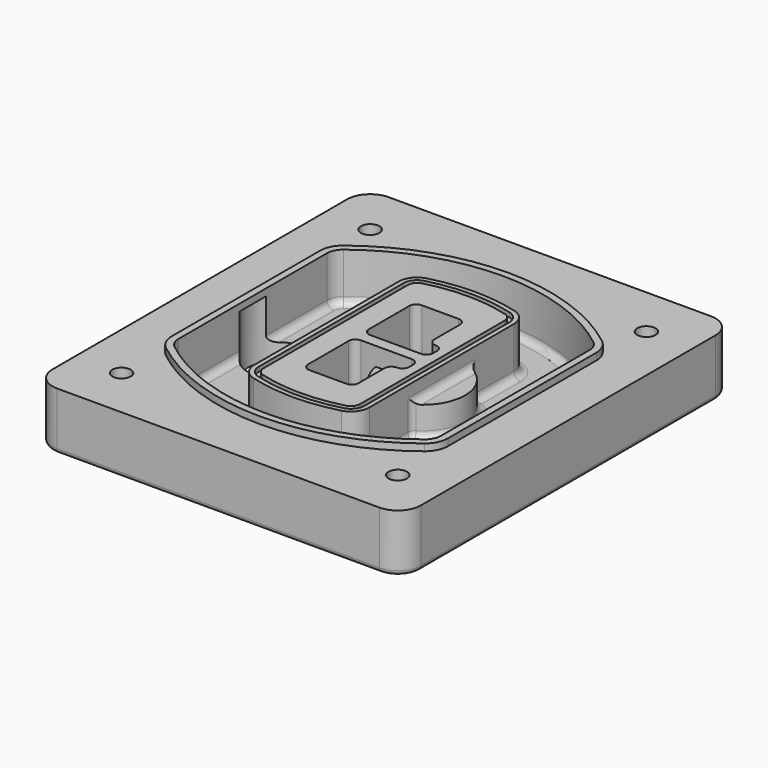
from build123d import *

# Parameters (mm, degrees)
F0_R      = 4
F1_DEPTH  = 25
F2_DEPTH  = 3
F3_DEPTH  = 18
F5_DEPTH  = 21
F6_DEPTH  = 2
F8_DEPTH  = 20
F9_DEPTH  = 16
F10_DEPTH = 25
F7_R      = 6
F7_R_2    = 4
F11_DEPTH = 6
F13_DEPTH = 9
F14_R     = 3
F15_R     = 2


# Not quite as in the source:
# - a feature of the source that left no trace in its solid (it failed there, or was rolled back) is left out


with BuildPart() as f1:
    # F0 (on Top) → F1 (new body)
    with BuildSketch(Plane.XY):
        with BuildLine():
            ThreePointArc((-80, -80), (-77.0710678119, -87.0710678119), (-70, -90))
            Line((-70, -90), (70, -90))
            ThreePointArc((70, -90), (77.0710678119, -87.0710678119), (80, -80))
            Line((80, -80), (80, 80))
            ThreePointArc((80, 80), (77.0710678119, 87.0710678119), (70, 90))
            Line((70, 90), (-70, 90))
            ThreePointArc((-70, 90), (-77.0710678119, 87.0710678119), (-80, 80))
            Line((-80, 80), (-80, -80))
        make_face()
        with Locations((-60, -67.5)):
            Circle(F0_R, mode=Mode.SUBTRACT)
        with Locations((60, -67.5)):
            Circle(F0_R, mode=Mode.SUBTRACT)
        with Locations((-60, 67.5)):
            Circle(F0_R, mode=Mode.SUBTRACT)
        with BuildLine():
            ThreePointArc((-64, 40.2934422872), (-62.5820384798, 46.4328484224), (-58.6153846154, 51.3286200352))
            ThreePointArc((-58.6153846154, 51.3286200352), (0, 71.5), (58.6153846154, 51.3286200352))
            ThreePointArc((58.6153846154, 51.3286200352), (62.5820384798, 46.4328484224), (64, 40.2934422872))
            Line((64, 40.2934422872), (64, -40.2934422872))
            ThreePointArc((64, -40.2934422872), (62.5820384798, -46.4328484224), (58.6153846154, -51.3286200352))
            ThreePointArc((58.6153846154, -51.3286200352), (0, -71.5), (-58.6153846154, -51.3286200352))
            ThreePointArc((-58.6153846154, -51.3286200352), (-62.5820384798, -46.4328484224), (-64, -40.2934422872))
            Line((-64, -40.2934422872), (-64, 40.2934422872))
        make_face(mode=Mode.SUBTRACT)
        with Locations((60, 67.5)):
            Circle(F0_R, mode=Mode.SUBTRACT)
        with BuildLine():
            ThreePointArc((58.6153846154, 51.3286200352), (0, 71.5), (-58.6153846154, 51.3286200352))
            ThreePointArc((-58.6153846154, 51.3286200352), (-62.5820384798, 46.4328484224), (-64, 40.2934422872))
            Line((-64, 40.2934422872), (-64, -40.2934422872))
            ThreePointArc((-64, -40.2934422872), (-62.5820384798, -46.4328484224), (-58.6153846154, -51.3286200352))
            ThreePointArc((-58.6153846154, -51.3286200352), (0, -71.5), (58.6153846154, -51.3286200352))
            ThreePointArc((58.6153846154, -51.3286200352), (62.5820384798, -46.4328484224), (64, -40.2934422872))
            Line((64, -40.2934422872), (64, 40.2934422872))
            ThreePointArc((64, 40.2934422872), (62.5820384798, 46.4328484224), (58.6153846154, 51.3286200352))
        make_face()
        with BuildLine():
            Line((-60, -40.2934422872), (-60, 40.2934422872))
            ThreePointArc((-60, 40.2934422872), (-58.9871703427, 44.6787323838), (-56.1538461538, 48.1757121072))
            ThreePointArc((-56.1538461538, 48.1757121072), (0, 67.5), (56.1538461538, 48.1757121072))
            ThreePointArc((56.1538461538, 48.1757121072), (58.9871703427, 44.6787323838), (60, 40.2934422872))
            Line((60, 40.2934422872), (60, -40.2934422872))
            ThreePointArc((60, -40.2934422872), (58.9871703427, -44.6787323838), (56.1538461538, -48.1757121072))
            ThreePointArc((56.1538461538, -48.1757121072), (0, -67.5), (-56.1538461538, -48.1757121072))
            ThreePointArc((-56.1538461538, -48.1757121072), (-58.9871703427, -44.6787323838), (-60, -40.2934422872))
        make_face(mode=Mode.SUBTRACT)
        with BuildLine():
            ThreePointArc((-56.1538461538, 48.1757121072), (-58.9871703427, 44.6787323838), (-60, 40.2934422872))
            Line((-60, 40.2934422872), (-60, -40.2934422872))
            ThreePointArc((-60, -40.2934422872), (-58.9871703427, -44.6787323838), (-56.1538461538, -48.1757121072))
            ThreePointArc((-56.1538461538, -48.1757121072), (0, -67.5), (56.1538461538, -48.1757121072))
            ThreePointArc((56.1538461538, -48.1757121072), (58.9871703427, -44.6787323838), (60, -40.2934422872))
            Line((60, -40.2934422872), (60, 40.2934422872))
            ThreePointArc((60, 40.2934422872), (58.9871703427, 44.6787323838), (56.1538461538, 48.1757121072))
            ThreePointArc((56.1538461538, 48.1757121072), (0, 67.5), (-56.1538461538, 48.1757121072))
        make_face()
        with BuildLine():
            ThreePointArc((54.3076923077, 45.8110311612), (56.2910192399, 43.3631453548), (57, 40.2934422872))
            Line((57, 40.2934422872), (57, -40.2934422872))
            ThreePointArc((57, -40.2934422872), (56.2910192399, -43.3631453548), (54.3076923077, -45.8110311612))
            ThreePointArc((54.3076923077, -45.8110311612), (0, -64.5), (-54.3076923077, -45.8110311612))
            ThreePointArc((-54.3076923077, -45.8110311612), (-56.2910192399, -43.3631453548), (-57, -40.2934422872))
            Line((-57, -40.2934422872), (-57, 40.2934422872))
            ThreePointArc((-57, 40.2934422872), (-56.2910192399, 43.3631453548), (-54.3076923077, 45.8110311612))
            ThreePointArc((-54.3076923077, 45.8110311612), (0, 64.5), (54.3076923077, 45.8110311612))
        make_face(mode=Mode.SUBTRACT)
        with BuildLine():
            Line((57, -40.2934422872), (57, 40.2934422872))
            ThreePointArc((57, 40.2934422872), (56.2910192399, 43.3631453548), (54.3076923077, 45.8110311612))
            ThreePointArc((54.3076923077, 45.8110311612), (0, 64.5), (-54.3076923077, 45.8110311612))
            ThreePointArc((-54.3076923077, 45.8110311612), (-56.2910192399, 43.3631453548), (-57, 40.2934422872))
            Line((-57, 40.2934422872), (-57, -40.2934422872))
            ThreePointArc((-57, -40.2934422872), (-56.2910192399, -43.3631453548), (-54.3076923077, -45.8110311612))
            ThreePointArc((-54.3076923077, -45.8110311612), (0, -64.5), (54.3076923077, -45.8110311612))
            ThreePointArc((54.3076923077, -45.8110311612), (56.2910192399, -43.3631453548), (57, -40.2934422872))
        make_face()
    extrude(amount=-F1_DEPTH)

    # F0 (on Top) → F2 (join)
    with BuildSketch(Plane.XY):
        with BuildLine():
            ThreePointArc((-56.1538461538, 48.1757121072), (-58.9871703427, 44.6787323838), (-60, 40.2934422872))
            Line((-60, 40.2934422872), (-60, -40.2934422872))
            ThreePointArc((-60, -40.2934422872), (-58.9871703427, -44.6787323838), (-56.1538461538, -48.1757121072))
            ThreePointArc((-56.1538461538, -48.1757121072), (0, -67.5), (56.1538461538, -48.1757121072))
            ThreePointArc((56.1538461538, -48.1757121072), (58.9871703427, -44.6787323838), (60, -40.2934422872))
            Line((60, -40.2934422872), (60, 40.2934422872))
            ThreePointArc((60, 40.2934422872), (58.9871703427, 44.6787323838), (56.1538461538, 48.1757121072))
            ThreePointArc((56.1538461538, 48.1757121072), (0, 67.5), (-56.1538461538, 48.1757121072))
        make_face()
        with BuildLine():
            ThreePointArc((54.3076923077, 45.8110311612), (56.2910192399, 43.3631453548), (57, 40.2934422872))
            Line((57, 40.2934422872), (57, -40.2934422872))
            ThreePointArc((57, -40.2934422872), (56.2910192399, -43.3631453548), (54.3076923077, -45.8110311612))
            ThreePointArc((54.3076923077, -45.8110311612), (0, -64.5), (-54.3076923077, -45.8110311612))
            ThreePointArc((-54.3076923077, -45.8110311612), (-56.2910192399, -43.3631453548), (-57, -40.2934422872))
            Line((-57, -40.2934422872), (-57, 40.2934422872))
            ThreePointArc((-57, 40.2934422872), (-56.2910192399, 43.3631453548), (-54.3076923077, 45.8110311612))
            ThreePointArc((-54.3076923077, 45.8110311612), (0, 64.5), (54.3076923077, 45.8110311612))
        make_face(mode=Mode.SUBTRACT)
    extrude(amount=F2_DEPTH)

    # F0 (on Top) → F3 (cut)
    with BuildSketch(Plane.XY):
        with BuildLine():
            Line((57, -40.2934422872), (57, 40.2934422872))
            ThreePointArc((57, 40.2934422872), (56.2910192399, 43.3631453548), (54.3076923077, 45.8110311612))
            ThreePointArc((54.3076923077, 45.8110311612), (0, 64.5), (-54.3076923077, 45.8110311612))
            ThreePointArc((-54.3076923077, 45.8110311612), (-56.2910192399, 43.3631453548), (-57, 40.2934422872))
            Line((-57, 40.2934422872), (-57, -40.2934422872))
            ThreePointArc((-57, -40.2934422872), (-56.2910192399, -43.3631453548), (-54.3076923077, -45.8110311612))
            ThreePointArc((-54.3076923077, -45.8110311612), (0, -64.5), (54.3076923077, -45.8110311612))
            ThreePointArc((54.3076923077, -45.8110311612), (56.2910192399, -43.3631453548), (57, -40.2934422872))
        make_face()
    extrude(amount=-F3_DEPTH, mode=Mode.SUBTRACT)

    # F4 (on face) → F5 (join, through all)
    with BuildSketch(Plane.XY.offset(3)):
        with BuildLine():
            ThreePointArc((-25, -39.2465276821), (-23.3511545998, -44.1109737193), (-19.0842911877, -46.9702398883))
            ThreePointArc((-19.0842911877, -46.9702398883), (0, -49.5), (19.0842911877, -46.9702398883))
            ThreePointArc((19.0842911877, -46.9702398883), (23.3511545998, -44.1109737193), (25, -39.2465276821))
            Line((25, -39.2465276821), (25, 39.2465276821))
            ThreePointArc((25, 39.2465276821), (23.3511545998, 44.1109737193), (19.0842911877, 46.9702398883))
            ThreePointArc((19.0842911877, 46.9702398883), (0, 49.5), (-19.0842911877, 46.9702398883))
            ThreePointArc((-19.0842911877, 46.9702398883), (-23.3511545998, 44.1109737193), (-25, 39.2465276821))
            Line((-25, 39.2465276821), (-25, -39.2465276821))
        make_face()
        with BuildLine():
            ThreePointArc((18.5632183908, 45.0393118368), (21.7633659499, 42.89486221), (23, 39.2465276821))
            Line((23, 39.2465276821), (23, -39.2465276821))
            ThreePointArc((23, -39.2465276821), (21.7633659499, -42.89486221), (18.5632183908, -45.0393118368))
            ThreePointArc((18.5632183908, -45.0393118368), (0, -47.5), (-18.5632183908, -45.0393118368))
            ThreePointArc((-18.5632183908, -45.0393118368), (-21.7633659499, -42.89486221), (-23, -39.2465276821))
            Line((-23, -39.2465276821), (-23, 39.2465276821))
            ThreePointArc((-23, 39.2465276821), (-21.7633659499, 42.89486221), (-18.5632183908, 45.0393118368))
            ThreePointArc((-18.5632183908, 45.0393118368), (0, 47.5), (18.5632183908, 45.0393118368))
        make_face(mode=Mode.SUBTRACT)
        with BuildLine():
            Line((23, -39.2465276821), (23, 39.2465276821))
            ThreePointArc((23, 39.2465276821), (21.7633659499, 42.89486221), (18.5632183908, 45.0393118368))
            ThreePointArc((18.5632183908, 45.0393118368), (0, 47.5), (-18.5632183908, 45.0393118368))
            ThreePointArc((-18.5632183908, 45.0393118368), (-21.7633659499, 42.89486221), (-23, 39.2465276821))
            Line((-23, 39.2465276821), (-23, -39.2465276821))
            ThreePointArc((-23, -39.2465276821), (-21.7633659499, -42.89486221), (-18.5632183908, -45.0393118368))
            ThreePointArc((-18.5632183908, -45.0393118368), (0, -47.5), (18.5632183908, -45.0393118368))
            ThreePointArc((18.5632183908, -45.0393118368), (21.7633659499, -42.89486221), (23, -39.2465276821))
        make_face()
        with BuildLine():
            ThreePointArc((18.0421455939, 43.1083837852), (20.1755772999, 41.6787507007), (21, 39.2465276821))
            Line((21, 39.2465276821), (21, -39.2465276821))
            ThreePointArc((21, -39.2465276821), (20.1755772999, -41.6787507007), (18.0421455939, -43.1083837852))
            ThreePointArc((18.0421455939, -43.1083837852), (0, -45.5), (-18.0421455939, -43.1083837852))
            ThreePointArc((-18.0421455939, -43.1083837852), (-20.1755772999, -41.6787507007), (-21, -39.2465276821))
            Line((-21, -39.2465276821), (-21, 39.2465276821))
            ThreePointArc((-21, 39.2465276821), (-20.1755772999, 41.6787507007), (-18.0421455939, 43.1083837852))
            ThreePointArc((-18.0421455939, 43.1083837852), (0, 45.5), (18.0421455939, 43.1083837852))
        make_face(mode=Mode.SUBTRACT)
        with BuildLine():
            Line((21, -39.2465276821), (21, 39.2465276821))
            ThreePointArc((21, 39.2465276821), (20.1755772999, 41.6787507007), (18.0421455939, 43.1083837852))
            ThreePointArc((18.0421455939, 43.1083837852), (0, 45.5), (-18.0421455939, 43.1083837852))
            ThreePointArc((-18.0421455939, 43.1083837852), (-20.1755772999, 41.6787507007), (-21, 39.2465276821))
            Line((-21, 39.2465276821), (-21, -39.2465276821))
            ThreePointArc((-21, -39.2465276821), (-20.1755772999, -41.6787507007), (-18.0421455939, -43.1083837852))
            ThreePointArc((-18.0421455939, -43.1083837852), (0, -45.5), (18.0421455939, -43.1083837852))
            ThreePointArc((18.0421455939, -43.1083837852), (20.1755772999, -41.6787507007), (21, -39.2465276821))
        make_face()
        with BuildLine():
            Line((-8, -2.5), (14, -2.5))
            ThreePointArc((14, -2.5), (16.1213203436, -3.3786796564), (17, -5.5))
            Line((17, -5.5), (17, -7.5))
            ThreePointArc((17, -7.5), (16.1213203436, -9.6213203436), (14, -10.5))
            ThreePointArc((14, -10.5), (11.8786796564, -11.3786796564), (11, -13.5))
            Line((11, -13.5), (11, -27.5))
            ThreePointArc((11, -27.5), (10.1213203436, -29.6213203436), (8, -30.5))
            Line((8, -30.5), (-8, -30.5))
            ThreePointArc((-8, -30.5), (-10.1213203436, -29.6213203436), (-11, -27.5))
            Line((-11, -27.5), (-11, -5.5))
            ThreePointArc((-11, -5.5), (-10.1213203436, -3.3786796564), (-8, -2.5))
        make_face(mode=Mode.SUBTRACT)
        with BuildLine():
            ThreePointArc((-8, 2.5), (-10.1213203436, 3.3786796564), (-11, 5.5))
            Line((-11, 5.5), (-11, 27.5))
            ThreePointArc((-11, 27.5), (-10.1213203436, 29.6213203436), (-8, 30.5))
            Line((-8, 30.5), (8, 30.5))
            ThreePointArc((8, 30.5), (10.1213203436, 29.6213203436), (11, 27.5))
            Line((11, 27.5), (11, 13.5))
            ThreePointArc((11, 13.5), (11.8786796564, 11.3786796564), (14, 10.5))
            ThreePointArc((14, 10.5), (16.1213203436, 9.6213203436), (17, 7.5))
            Line((17, 7.5), (17, 5.5))
            ThreePointArc((17, 5.5), (16.1213203436, 3.3786796564), (14, 2.5))
            Line((14, 2.5), (-8, 2.5))
        make_face(mode=Mode.SUBTRACT)
    extrude(amount=-F5_DEPTH)

    # F4 (on face) → F6 (cut)
    with BuildSketch(Plane.XY.offset(3)):
        with BuildLine():
            Line((23, -39.2465276821), (23, 39.2465276821))
            ThreePointArc((23, 39.2465276821), (21.7633659499, 42.89486221), (18.5632183908, 45.0393118368))
            ThreePointArc((18.5632183908, 45.0393118368), (0, 47.5), (-18.5632183908, 45.0393118368))
            ThreePointArc((-18.5632183908, 45.0393118368), (-21.7633659499, 42.89486221), (-23, 39.2465276821))
            Line((-23, 39.2465276821), (-23, -39.2465276821))
            ThreePointArc((-23, -39.2465276821), (-21.7633659499, -42.89486221), (-18.5632183908, -45.0393118368))
            ThreePointArc((-18.5632183908, -45.0393118368), (0, -47.5), (18.5632183908, -45.0393118368))
            ThreePointArc((18.5632183908, -45.0393118368), (21.7633659499, -42.89486221), (23, -39.2465276821))
        make_face()
        with BuildLine():
            ThreePointArc((18.0421455939, 43.1083837852), (20.1755772999, 41.6787507007), (21, 39.2465276821))
            Line((21, 39.2465276821), (21, -39.2465276821))
            ThreePointArc((21, -39.2465276821), (20.1755772999, -41.6787507007), (18.0421455939, -43.1083837852))
            ThreePointArc((18.0421455939, -43.1083837852), (0, -45.5), (-18.0421455939, -43.1083837852))
            ThreePointArc((-18.0421455939, -43.1083837852), (-20.1755772999, -41.6787507007), (-21, -39.2465276821))
            Line((-21, -39.2465276821), (-21, 39.2465276821))
            ThreePointArc((-21, 39.2465276821), (-20.1755772999, 41.6787507007), (-18.0421455939, 43.1083837852))
            ThreePointArc((-18.0421455939, 43.1083837852), (0, 45.5), (18.0421455939, 43.1083837852))
        make_face(mode=Mode.SUBTRACT)
    extrude(amount=-F6_DEPTH, mode=Mode.SUBTRACT)

    # F7 (on face) → F8 (join)
    with BuildSketch(Plane(origin=(0, 0, -25), x_dir=(1, 0, 0), z_dir=(0, 0, -1))):
        with BuildLine():
            ThreePointArc((3.28842436, 0), (16.7567035675, 13.4682792075), (30.224982775, 0))
            Line((30.224982775, 0), (35.224982775, 0))
            ThreePointArc((35.224982775, 0), (16.7567035675, 18.4682792075), (-1.71157564, 0))
            Line((-1.71157564, 0), (3.28842436, 0))
        make_face()
        with BuildLine():
            Line((3.28842436, 0), (30.224982775, 0))
            ThreePointArc((30.224982775, 0), (16.7567035675, 13.4682792075), (3.28842436, 0))
        make_face()
        with BuildLine():
            ThreePointArc((3.28842436, 0), (16.7567035675, -13.4682792075), (30.224982775, 0))
            Line((30.224982775, 0), (3.28842436, 0))
        make_face()
        with BuildLine():
            Line((35.224982775, 0), (30.224982775, 0))
            ThreePointArc((30.224982775, 0), (16.7567035675, -13.4682792075), (3.28842436, 0))
            Line((3.28842436, 0), (-1.71157564, 0))
            ThreePointArc((-1.71157564, 0), (16.7567035675, -18.4682792075), (35.224982775, 0))
        make_face()
    extrude(amount=-F8_DEPTH)

    # F7 (on face) → F9 (cut)
    with BuildSketch(Plane(origin=(0, 0, -25), x_dir=(1, 0, 0), z_dir=(0, 0, -1))):
        with BuildLine():
            Line((3.28842436, 0), (30.224982775, 0))
            ThreePointArc((30.224982775, 0), (16.7567035675, 13.4682792075), (3.28842436, 0))
        make_face()
        with BuildLine():
            ThreePointArc((3.28842436, 0), (16.7567035675, -13.4682792075), (30.224982775, 0))
            Line((30.224982775, 0), (3.28842436, 0))
        make_face()
    extrude(amount=-F9_DEPTH, mode=Mode.SUBTRACT)

    # F7 (on face) → F10 (cut)
    with BuildSketch(Plane(origin=(0, 0, -25), x_dir=(1, 0, 0), z_dir=(0, 0, -1))):
        with BuildLine():
            Line((-59.0318229325, 0), (-32.0952645175, 0))
            ThreePointArc((-32.0952645175, 0), (-45.563543725, 13.4682792075), (-59.0318229325, 0))
        make_face()
        with BuildLine():
            ThreePointArc((-59.0318229325, 0), (-45.563543725, -13.4682792075), (-32.0952645175, 0))
            Line((-32.0952645175, 0), (-59.0318229325, 0))
        make_face()
    extrude(amount=-F10_DEPTH, mode=Mode.SUBTRACT)

    # F7 (on face) → F11 (cut)
    with BuildSketch(Plane(origin=(0, 0, -25), x_dir=(1, 0, 0), z_dir=(0, 0, -1))):
        with Locations((60, -67.5)):
            Circle(F7_R)
        with Locations((60, -67.5)):
            Circle(F7_R_2, mode=Mode.SUBTRACT)
        with Locations((-60, -67.5)):
            Circle(F7_R)
        with Locations((-60, -67.5)):
            Circle(F7_R_2, mode=Mode.SUBTRACT)
        with Locations((-60, 67.5)):
            Circle(F7_R)
        with Locations((-60, 67.5)):
            Circle(F7_R_2, mode=Mode.SUBTRACT)
        with Locations((60, 67.5)):
            Circle(F7_R)
        with Locations((60, 67.5)):
            Circle(F7_R_2, mode=Mode.SUBTRACT)
    extrude(amount=-F11_DEPTH, mode=Mode.SUBTRACT)

    # F12 (on face) → F13 (cut, through all)
    with BuildSketch(Plane(origin=(0, 0, -9), x_dir=(1, 0, 0), z_dir=(0, 0, -1))):
        with BuildLine():
            Line((11, 13.5), (11, 17.5481537753))
            ThreePointArc((11, 17.5481537753), (2.5696536419, 11.8239143813), (-1.5415842455, 2.5))
            Line((-1.5415842455, 2.5), (3.5224848595, 2.5))
            ThreePointArc((3.5224848595, 2.5), (6.1857188154, 8.3455872281), (11.2536447004, 12.2927168648))
            ThreePointArc((11.2536447004, 12.2927168648), (11.0640958889, 12.8831798879), (11, 13.5))
        make_face()
        with BuildLine():
            ThreePointArc((11.2536447004, -12.2927168648), (6.1857188154, -8.3455872281), (3.5224848595, -2.5))
            Line((3.5224848595, -2.5), (-1.5415842455, -2.5))
            ThreePointArc((-1.5415842455, -2.5), (2.5696536419, -11.8239143813), (11, -17.5481537753))
            Line((11, -17.5481537753), (11, -13.5))
            ThreePointArc((11, -13.5), (11.0640958889, -12.8831798879), (11.2536447004, -12.2927168648))
        make_face()
        with BuildLine():
            ThreePointArc((11.2536447004, 12.2927168648), (6.1857188154, 8.3455872281), (3.5224848595, 2.5))
            Line((3.5224848595, 2.5), (14, 2.5))
            ThreePointArc((14, 2.5), (16.1213203436, 3.3786796564), (17, 5.5))
            Line((17, 5.5), (17, 7.5))
            ThreePointArc((17, 7.5), (16.1213203436, 9.6213203436), (14, 10.5))
            ThreePointArc((14, 10.5), (12.3601599782, 10.9878446101), (11.2536447004, 12.2927168648))
        make_face()
        with BuildLine():
            Line((14, -2.5), (3.5224848595, -2.5))
            ThreePointArc((3.5224848595, -2.5), (6.1857188154, -8.3455872281), (11.2536447004, -12.2927168648))
            ThreePointArc((11.2536447004, -12.2927168648), (12.3601599782, -10.9878446101), (14, -10.5))
            ThreePointArc((14, -10.5), (16.1213203436, -9.6213203436), (17, -7.5))
            Line((17, -7.5), (17, -5.5))
            ThreePointArc((17, -5.5), (16.1213203436, -3.3786796564), (14, -2.5))
        make_face()
    extrude(amount=F13_DEPTH, mode=Mode.SUBTRACT)

    # F14
    f14_edges = [f1.edges().sort_by_distance(p)[0] for p in [
        (-57, -23.703476, -18),
        (-57, 23.703476, -18),
        (25, 0, -5),
        (25, 16.526506, -11.5),
        (25, -16.526506, -11.5),
        (25, -27.886517, -18),
        (35.224983, 0, -18),
        (23.351155, -44.110974, -18),
        (-56.291019, -43.363145, -18),
        (-56.291019, 43.363145, -18),
        (0, 64.5, -18),
        (56.291019, 43.363145, -18),
        (57, 0, -18),
        (56.291019, -43.363145, -18),
        (0, -64.5, -18),
        (-23.351155, 44.110974, -18),
        (0, 49.5, -18),
        (-25, 0, -18),
        (23.351155, 44.110974, -18),
        (-23.351155, -44.110974, -18),
        (25, 27.886517, -18),
        (0, -49.5, -18),
    ]]
    fillet(f14_edges, radius=F14_R)

    # F15
    f15_edges = [f1.edges().sort_by_distance(p)[0] for p in [
        (0, -90, -25),
        (-77.071068, -87.071068, -25),
        (-80, 0, -25),
        (-77.071068, 87.071068, -25),
        (77.071068, -87.071068, -25),
        (0, 90, -25),
        (80, 0, -25),
        (77.071068, 87.071068, -25),
    ]]
    fillet(f15_edges, radius=F15_R)


solid = f1.part
